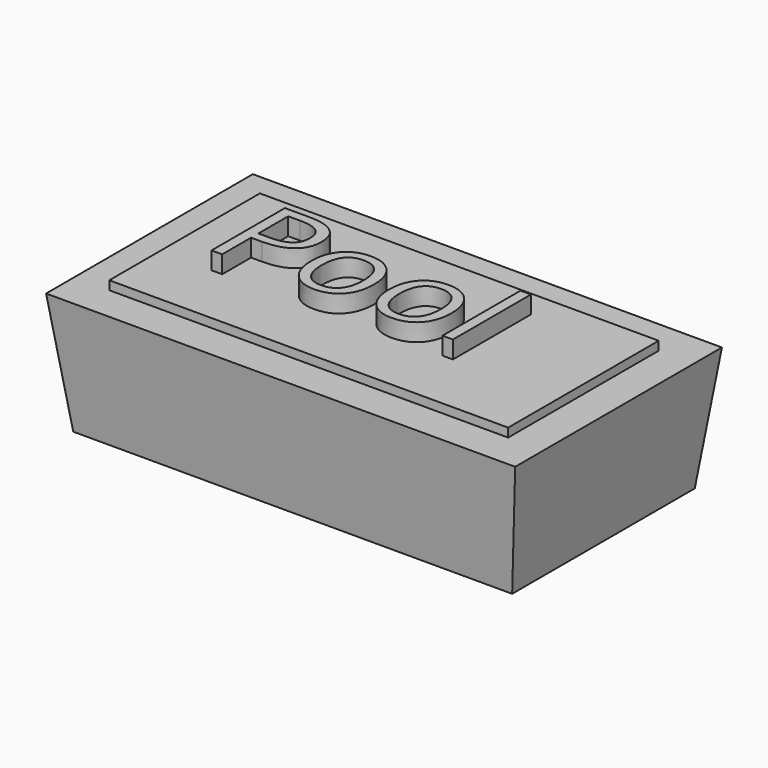
from build123d import *

# Parameters (mm, degrees)
F0_W         = 2500
F0_H         = 1300
F1_DEPTH     = 700
F1_TAPER     = -7
F2_W         = 2271.8983852641
F2_H         = 1071.8983852641
F3_DEPTH     = 50
F4_TEXT_SIZE = 731.4951469501
F5_DEPTH     = 100


# Not quite as in the source:
# - Text() gives the source's letters only with a copy of the font that has no kerning and outlines rounded to 1/6400 em; it was checked with that copy


with BuildPart() as f1:
    # F0 (on Top) → F1 (new body)
    with BuildSketch(Plane.XY):
        Rectangle(F0_W, F0_H)
    extrude(amount=F1_DEPTH, taper=F1_TAPER)


with BuildPart() as f3:
    # F2 (on face) → F3 (new body)
    with BuildSketch(Plane.XY.offset(700)):
        Rectangle(F2_W, F2_H)
    extrude(amount=F3_DEPTH)


with BuildPart() as f5:
    # F4 (on face) → F5 (new body)
    with BuildSketch(Plane.XY.offset(750)):
        with Locations((-912.3303294182, -176.9978404045)):
            Text('Pool', F4_TEXT_SIZE, font='Open Sans', text_align=(TextAlign.LEFT, TextAlign.BOTTOM))
    extrude(amount=F5_DEPTH)


solid = Compound([f1.part, f3.part, f5.part])
